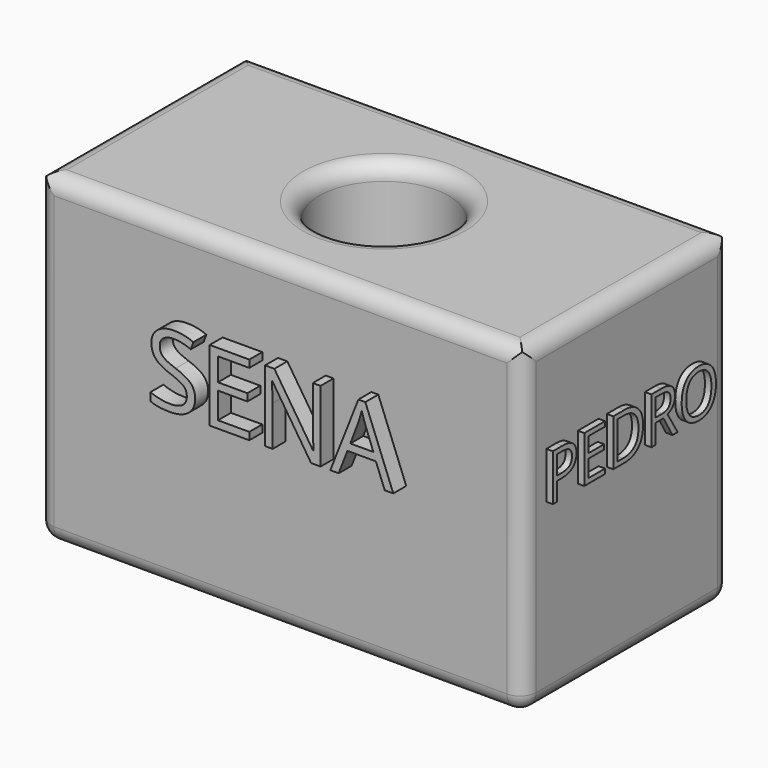
from build123d import *

# Parameters (mm, degrees)
F0_W         = 150
F0_H         = 100
F1_DEPTH     = 40
F2_R         = 20
F3_DEPTH     = 74
F4_R         = 5
F5_T1_DEPTH  = 102.5
F5_T3_DEPTH  = 140
F5_T5_DEPTH  = 70
F5_S9_W      = 5.1
F5_S9_H      = 5.1
F5_T10_DEPTH = 5.1
F5_S15_W     = 5.1
F5_S15_H     = 5.1
F5_T16_DEPTH = 5.1
F5_S21_W     = 5.1
F5_S21_H     = 5.1
F5_T22_DEPTH = 5.1
F5_S27_W     = 5.1
F5_S27_H     = 5.1
F5_T28_DEPTH = 5.1
F6_TEXT_SIZE = 30.7459701111
F7_DEPTH     = 5
F8_TEXT_SIZE = 20.1612904978
F9_DEPTH     = 2


# Not quite as in the source:
# - a fillet or chamfer that OpenCascade refuses, or shapes differently, is made with other operations: its cross-section is extruded or revolved along the edge and cut away or added
# - Text() gives the source's letters only with a copy of the font that has no kerning and outlines rounded to 1/6400 em; it was checked with that copy


with BuildPart() as f1:
    # F0 (on Front) → F1 (new body, symmetric)
    with BuildSketch(Plane.XZ):
        Rectangle(F0_W, F0_H)
    extrude(amount=F1_DEPTH, both=True)

    # F2 (on Top) → F3 (cut, symmetric)
    with BuildSketch(Plane.XY):
        Circle(F2_R)
    extrude(amount=F3_DEPTH, both=True, mode=Mode.SUBTRACT)

    # F4
    f4_edges = [f1.edges().sort_by_distance(p)[0] for p in [
        (75, 0, 50),
        (0, 40, 50),
        (0, -40, 50),
        (-75, 0, 50),
        (-20, 0, 50),
    ]]
    fillet(f4_edges, radius=F4_R)

    # F5: fillet of radius 5 on 12 edges, made by hand

    # F5_s2 → F5_t1 (cut)
    with BuildSketch(Plane.XY.offset(-45)):
        with BuildLine():
            ThreePointArc((75, -35), (73.5355339059, -38.5355339059), (70, -40))
            Line((70, -40), (75, -40))
            Line((75, -40), (75, -35))
        make_face()
        with BuildLine():
            ThreePointArc((-70, -40), (-73.5355339059, -38.5355339059), (-75, -35))
            Line((-75, -35), (-75, -40))
            Line((-75, -40), (-70, -40))
        make_face()
        with BuildLine():
            ThreePointArc((-70, 40), (-73.5355339059, 38.5355339059), (-75, 35))
            Line((-75, 35), (-75, 40))
            Line((-75, 40), (-70, 40))
        make_face()
        with BuildLine():
            ThreePointArc((75, 35), (73.5355339059, 38.5355339059), (70, 40))
            Line((70, 40), (75, 40))
            Line((75, 40), (75, 35))
        make_face()
    extrude(amount=F5_T1_DEPTH, mode=Mode.SUBTRACT)

    # F5_s4 → F5_t3 (cut)
    with BuildSketch(Plane.YZ.offset(-70)):
        with BuildLine():
            ThreePointArc((-35, -50), (-38.5355339059, -48.5355339059), (-40, -45))
            Line((-40, -45), (-40, -50))
            Line((-40, -50), (-35, -50))
        make_face()
        with BuildLine():
            ThreePointArc((40, -45), (38.5355339059, -48.5355339059), (35, -50))
            Line((35, -50), (40, -50))
            Line((40, -50), (40, -45))
        make_face()
    extrude(amount=F5_T3_DEPTH, mode=Mode.SUBTRACT)

    # F5_s6 → F5_t5 (cut)
    with BuildSketch(Plane.XZ.offset(-35)):
        with BuildLine():
            ThreePointArc((-70, -50), (-73.5355339059, -48.5355339059), (-75, -45))
            Line((-75, -45), (-75, -50))
            Line((-75, -50), (-70, -50))
        make_face()
        with BuildLine():
            ThreePointArc((75, -45), (73.5355339059, -48.5355339059), (70, -50))
            Line((70, -50), (75, -50))
            Line((75, -50), (75, -45))
        make_face()
    extrude(amount=F5_T5_DEPTH, mode=Mode.SUBTRACT)


with BuildPart() as f5_tool8:
    # F5_s9 → F5_t10 (new body)
    with BuildSketch(Plane.YZ.offset(70)):
        with Locations((-37.55, -47.55)):
            Rectangle(F5_S9_W, F5_S9_H)
    extrude(amount=F5_T10_DEPTH)

    # F5_s11 → F5_t12 (revolve, cut)
    with BuildSketch(Plane(origin=(70, -35, -45), x_dir=(0, 0.7071067812, 0.7071067812), z_dir=(0, 0.7071067812, -0.7071067812))):
        with BuildLine():
            ThreePointArc((0, -5), (5, 0), (0, 5))
            Line((0, 5), (0, -5))
        make_face()
    revolve(axis=Axis((70, -35, -45), (1, 0, 0)), mode=Mode.SUBTRACT)


with BuildPart() as f1_1:
    add(f1.part)

    # F5_t7: cut F5_tool8
    add(f5_tool8.part, mode=Mode.SUBTRACT)


with BuildPart() as f5_tool14:
    # F5_s15 → F5_t16 (new body)
    with BuildSketch(Plane.XY.offset(-45)):
        with Locations((-72.55, -37.55)):
            Rectangle(F5_S15_W, F5_S15_H)
    extrude(amount=-F5_T16_DEPTH)

    # F5_s17 → F5_t18 (revolve, cut)
    with BuildSketch(Plane(origin=(-70, -35, -45), x_dir=(0.7071067812, 0.7071067812, 0), z_dir=(-0.7071067812, 0.7071067812, 0))):
        with BuildLine():
            ThreePointArc((0, -5), (5, 0), (0, 5))
            Line((0, 5), (0, -5))
        make_face()
    revolve(axis=Axis((-70, -35, -45), (0, 0, -1)), mode=Mode.SUBTRACT)


with BuildPart() as f1_2:
    add(f1_1.part)

    # F5_t13: cut F5_tool14
    add(f5_tool14.part, mode=Mode.SUBTRACT)


with BuildPart() as f5_tool20:
    # F5_s21 → F5_t22 (new body)
    with BuildSketch(Plane.XZ.offset(-35)):
        with Locations((-72.55, -47.55)):
            Rectangle(F5_S21_W, F5_S21_H)
    extrude(amount=-F5_T22_DEPTH)

    # F5_s23 → F5_t24 (revolve, cut)
    with BuildSketch(Plane(origin=(-70, 35, -45), x_dir=(0.7071067812, 0, 0.7071067812), z_dir=(-0.7071067812, 0, 0.7071067812))):
        with BuildLine():
            ThreePointArc((0, -5), (5, 0), (0, 5))
            Line((0, 5), (0, -5))
        make_face()
    revolve(axis=Axis((-70, 35, -45), (0, 1, 0)), mode=Mode.SUBTRACT)


with BuildPart() as f1_3:
    add(f1_2.part)

    # F5_t19: cut F5_tool20
    add(f5_tool20.part, mode=Mode.SUBTRACT)


with BuildPart() as f5_tool26:
    # F5_s27 → F5_t28 (new body)
    with BuildSketch(Plane.YZ.offset(70)):
        with Locations((37.55, -47.55)):
            Rectangle(F5_S27_W, F5_S27_H)
    extrude(amount=F5_T28_DEPTH)

    # F5_s29 → F5_t30 (revolve, cut)
    with BuildSketch(Plane(origin=(70, 35, -45), x_dir=(0, -0.7071067812, 0.7071067812), z_dir=(0, 0.7071067812, 0.7071067812))):
        with BuildLine():
            ThreePointArc((0, -5), (5, 0), (0, 5))
            Line((0, 5), (0, -5))
        make_face()
    revolve(axis=Axis((70, 35, -45), (1, 0, 0)), mode=Mode.SUBTRACT)


with BuildPart() as f1_4:
    add(f1_3.part)

    # F5_t25: cut F5_tool26
    add(f5_tool26.part, mode=Mode.SUBTRACT)

    # F5_s31 → F5_t32 (revolve, cut)
    with BuildSketch(Plane.XZ):
        with BuildLine():
            ThreePointArc((25, -50), (21.4644660941, -48.5355339059), (20, -45))
            Line((20, -45), (20, -50))
            Line((20, -50), (25, -50))
        make_face()
    revolve(axis=Axis((0, 0, -50), (0, 0, 1)), mode=Mode.SUBTRACT)

    # F6 (on face) → F7 (join)
    with BuildSketch(Plane.XZ.offset(40)):
        with Locations((-37.7419367433, 1.4516129158)):
            Text('SENA', F6_TEXT_SIZE, font='Open Sans', text_align=(TextAlign.LEFT, TextAlign.BOTTOM))
    extrude(amount=F7_DEPTH)

    # F8 (on face) → F9 (join)
    with BuildSketch(Plane.YZ.offset(75)):
        with Locations((-33.024195116, 5.2620982751)):
            Text('PEDRO', F8_TEXT_SIZE, font='Open Sans', text_align=(TextAlign.LEFT, TextAlign.BOTTOM))
    extrude(amount=F9_DEPTH)


solid = f1_4.part
